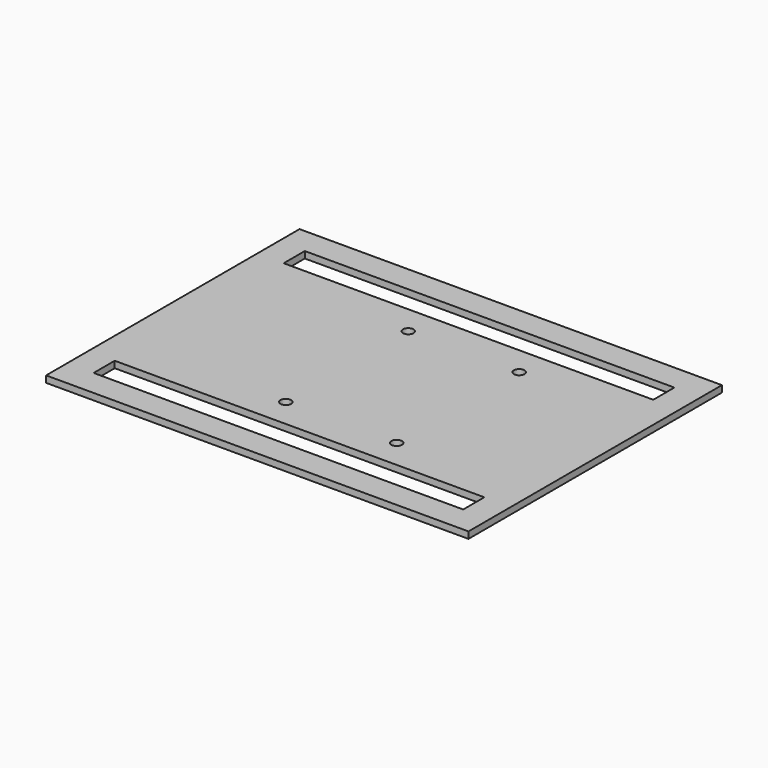
from build123d import *

# Parameters (mm, degrees)
F0_W     = 203.2
F0_H     = 152.4
F0_W_2   = 177.8
F0_H_2   = 12.7
F0_R     = 2.54
F1_DEPTH = 3.175


# Not quite as in the source:
# - a length typed as a fraction of an inch, garbled in the dataset ("3 / 203.2 mm" for 3/8 in), is restored
# - a feature names something its author has since deleted; it is built from what else it names


with BuildPart() as f1:
    # F0 (on Top) → F1 (new body)
    with BuildSketch(Plane.XY):
        Rectangle(F0_W, F0_H)
        with Locations((0, -57.15)):
            Rectangle(F0_W_2, F0_H_2, mode=Mode.SUBTRACT)
        with Locations((-17.78, -36.83)):
            Circle(F0_R, mode=Mode.SUBTRACT)
        with Locations((35.56, -36.83)):
            Circle(F0_R, mode=Mode.SUBTRACT)
        with Locations((-17.78, 36.83)):
            Circle(F0_R, mode=Mode.SUBTRACT)
        with Locations((0, 57.15)):
            Rectangle(F0_W_2, F0_H_2, mode=Mode.SUBTRACT)
        with Locations((35.56, 36.83)):
            Circle(F0_R, mode=Mode.SUBTRACT)
    extrude(amount=F1_DEPTH)


solid = f1.part
